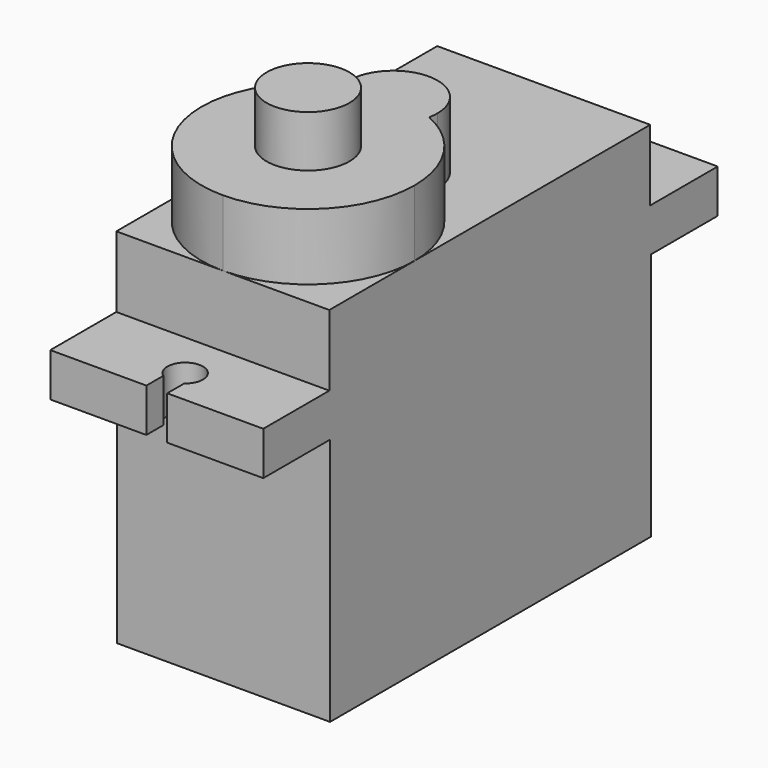
from build123d import *

# Parameters (mm, degrees)
F0_W     = 12
F0_H     = 22.6
F1_DEPTH = 14
F2_W     = 12
F2_H     = 22.6
F3_DEPTH = 2.45
F4_W     = 12
F4_H     = 22.6
F5_DEPTH = 4
F7_DEPTH = 3.74
F8_R     = 2.335
F9_DEPTH = 2.9


# Not quite as in the source:
# - a feature names something its author has since deleted; it is built from what else it names


with BuildPart() as f1:
    # F0 (on Top) → F1 (new body)
    with BuildSketch(Plane.XY):
        with Locations((13.4373875856, -22.2866622627)):
            Rectangle(F0_W, F0_H)
    extrude(amount=F1_DEPTH)

    # F2 (on face) → F3 (join)
    with BuildSketch(Plane.XY.offset(14)):
        with BuildLine():
            Line((7.4373875856, -10.9866622627), (19.4373875856, -10.9866622627))
            Line((19.4373875856, -10.9866622627), (19.4373875856, -6.2866622627))
            Line((19.4373875856, -6.2866622627), (14.0248552029, -6.2866622627))
            Line((14.0248552029, -6.2866622627), (14.0248552029, -7.4774145882))
            ThreePointArc((14.0248552029, -7.4774145882), (14.3283049828, -7.8324968838), (14.4373875856, -8.2866622627))
            ThreePointArc((14.4373875856, -8.2866622627), (12.9832222068, -9.1775796599), (12.8499199684, -7.4774145882))
            Line((12.8499199684, -7.4774145882), (12.8499199684, -6.2866622627))
            Line((12.8499199684, -6.2866622627), (7.4373875856, -6.2866622627))
            Line((7.4373875856, -6.2866622627), (7.4373875856, -10.9866622627))
        make_face()
        with BuildLine():
            Line((19.4373875856, -38.2866622627), (19.4373875856, -33.5866622627))
            Line((19.4373875856, -33.5866622627), (7.4373875856, -33.5866622627))
            Line((7.4373875856, -33.5866622627), (7.4373875856, -38.2866622627))
            Line((7.4373875856, -38.2866622627), (12.8499199684, -38.2866622627))
            Line((12.8499199684, -38.2866622627), (12.8499199684, -37.0959099372))
            ThreePointArc((12.8499199684, -37.0959099372), (12.9832222068, -35.3957448655), (14.4373875856, -36.2866622627))
            ThreePointArc((14.4373875856, -36.2866622627), (14.3283049828, -36.7408276416), (14.0248552029, -37.0959099372))
            Line((14.0248552029, -37.0959099372), (14.0248552029, -38.2866622627))
            Line((14.0248552029, -38.2866622627), (19.4373875856, -38.2866622627))
        make_face()
        with Locations((13.4373875856, -22.2866622627)):
            Rectangle(F2_W, F2_H)
    extrude(amount=F3_DEPTH)

    # F4 (on face) → F5 (join)
    with BuildSketch(Plane.XY.offset(16.45)):
        with Locations((13.4373875856, -22.3371585727)):
            Rectangle(F4_W, F4_H)
    extrude(amount=F5_DEPTH)

    # F6 (on face) → F7 (join)
    with BuildSketch(Plane.XY.offset(20.45)):
        with BuildLine():
            ThreePointArc((13.4373875856, -33.6371585727), (17.6800282728, -31.8797992598), (19.4373875856, -27.6371585727))
            ThreePointArc((19.4373875856, -27.6371585727), (18.4708192303, -24.371493881), (15.8825322928, -22.157991906))
            ThreePointArc((15.8825322928, -22.157991906), (13.4373875856, -24.1371585727), (10.9922428785, -22.157991906))
            ThreePointArc((10.9922428785, -22.157991906), (8.403955941, -24.371493881), (7.4373875856, -27.6371585727))
            ThreePointArc((7.4373875856, -27.6371585727), (9.1947468985, -31.8797992598), (13.4373875856, -33.6371585727))
        make_face()
        with BuildLine():
            ThreePointArc((10.9922428785, -22.157991906), (13.4373875856, -24.1371585727), (15.8825322928, -22.157991906))
            ThreePointArc((15.8825322928, -22.157991906), (13.4373875856, -21.6371585727), (10.9922428785, -22.157991906))
        make_face()
        with BuildLine():
            ThreePointArc((10.9922428785, -22.157991906), (13.4373875856, -21.6371585727), (15.8825322928, -22.157991906))
            ThreePointArc((15.8825322928, -22.157991906), (15.9236359409, -21.8990156254), (15.9373875856, -21.6371585727))
            ThreePointArc((15.9373875856, -21.6371585727), (13.1755305329, -19.1509102174), (10.9922428785, -22.157991906))
        make_face()
    extrude(amount=F7_DEPTH)

    # F8 (on face) → F9 (join)
    with BuildSketch(Plane.XY.offset(24.19)):
        with Locations((13.4373875856, -27.6371585727)):
            Circle(F8_R)
    extrude(amount=F9_DEPTH)


solid = f1.part
